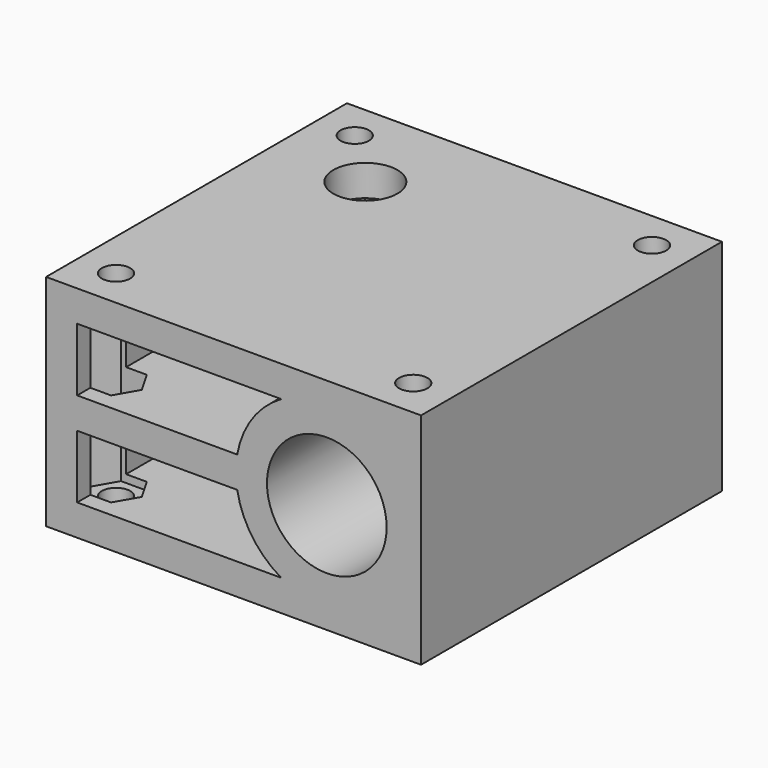
from build123d import *

# Parameters (mm, degrees)
F3_W          = 48.25
F3_H          = 28.25
F3_R          = 7.7
F4_DEPTH      = 24.2
F5_R          = 1.825
F6_DEPTH      = 28.25
F5_R_2        = 4.125
F7_DEPTH      = 28.25
F9_DEPTH      = 13.125
F9_DEPTH_BACK = 9.125


# Not quite as in the source:
# - a feature names something its author has since deleted; it is built from what else it names


with BuildPart() as f4:
    # F3 (on Front) → F4 (new body, symmetric)
    with BuildSketch(Plane.XZ):
        Rectangle(F3_W, F3_H)
        with BuildLine():
            ThreePointArc((23.5277925033, 2), (23.6568686252, 1.0037000824), (23.7, 0))
            ThreePointArc((23.7, 0), (23.6568686252, -1.0037000824), (23.5277925033, -2))
            ThreePointArc((23.5277925033, -2), (22.3372126342, -5.4801491728), (20.125, -8.4186920005))
            Line((20.125, -8.4186920005), (20.125, -10.125))
            Line((20.125, -10.125), (17.8629663994, -10.125))
            ThreePointArc((17.8629663994, -10.125), (15.9935594213, -10.9973398215), (14, -11.5277925033))
            ThreePointArc((14, -11.5277925033), (12, -11.7), (10, -11.5277925033))
            ThreePointArc((10, -11.5277925033), (8.0064405787, -10.9973398215), (6.1370336006, -10.125))
            Line((6.1370336006, -10.125), (-20.125, -10.125))
            Line((-20.125, -10.125), (-20.125, -2))
            Line((-20.125, -2), (-20.125, 2))
            Line((-20.125, 2), (-20.125, 10.125))
            Line((-20.125, 10.125), (6.1370336006, 10.125))
            ThreePointArc((6.1370336006, 10.125), (8.0064405787, 10.9973398215), (10, 11.5277925033))
            ThreePointArc((10, 11.5277925033), (12, 11.7), (14, 11.5277925033))
            ThreePointArc((14, 11.5277925033), (15.9935594213, 10.9973398215), (17.8629663994, 10.125))
            Line((17.8629663994, 10.125), (20.125, 10.125))
            Line((20.125, 10.125), (20.125, 8.4186920005))
            ThreePointArc((20.125, 8.4186920005), (22.3372126342, 5.4801491728), (23.5277925033, 2))
        make_face(mode=Mode.SUBTRACT)
        with BuildLine():
            Line((14, 10.125), (14, 11.5277925033))
            ThreePointArc((14, 11.5277925033), (12, 11.7), (10, 11.5277925033))
            Line((10, 11.5277925033), (10, 10.125))
            Line((10, 10.125), (14, 10.125))
        make_face()
        with BuildLine():
            Line((20.125, 2), (20.125, 8.4186920005))
            ThreePointArc((20.125, 8.4186920005), (19.045826619, 9.3405742466), (17.8629663994, 10.125))
            Line((17.8629663994, 10.125), (14, 10.125))
            Line((14, 10.125), (10, 10.125))
            Line((10, 10.125), (6.1370336006, 10.125))
            ThreePointArc((6.1370336006, 10.125), (2.4024206149, 6.6915222444), (0.4722074967, 2))
            ThreePointArc((0.4722074967, 2), (0.3, 0), (0.4722074967, -2))
            ThreePointArc((0.4722074967, -2), (2.4024206149, -6.6915222444), (6.1370336006, -10.125))
            Line((6.1370336006, -10.125), (10, -10.125))
            Line((10, -10.125), (14, -10.125))
            Line((14, -10.125), (17.8629663994, -10.125))
            ThreePointArc((17.8629663994, -10.125), (19.045826619, -9.3405742466), (20.125, -8.4186920005))
            Line((20.125, -8.4186920005), (20.125, -2))
            Line((20.125, -2), (20.125, 2))
        make_face()
        with Locations((12, 0)):
            Circle(F3_R, mode=Mode.SUBTRACT)
        with BuildLine():
            ThreePointArc((10, -11.5277925033), (12, -11.7), (14, -11.5277925033))
            Line((14, -11.5277925033), (14, -10.125))
            Line((14, -10.125), (10, -10.125))
            Line((10, -10.125), (10, -11.5277925033))
        make_face()
        with BuildLine():
            ThreePointArc((0.4722074967, -2), (0.3, 0), (0.4722074967, 2))
            Line((0.4722074967, 2), (-20.125, 2))
            Line((-20.125, 2), (-20.125, -2))
            Line((-20.125, -2), (0.4722074967, -2))
        make_face()
        with BuildLine():
            ThreePointArc((23.5277925033, -2), (23.6568686252, -1.0037000824), (23.7, 0))
            ThreePointArc((23.7, 0), (23.6568686252, 1.0037000824), (23.5277925033, 2))
            Line((23.5277925033, 2), (20.125, 2))
            Line((20.125, 2), (20.125, -2))
            Line((20.125, -2), (23.5277925033, -2))
        make_face()
        with BuildLine():
            Line((20.125, 2), (23.5277925033, 2))
            ThreePointArc((23.5277925033, 2), (22.3372126342, 5.4801491728), (20.125, 8.4186920005))
            Line((20.125, 8.4186920005), (20.125, 2))
        make_face()
        with BuildLine():
            ThreePointArc((20.125, -8.4186920005), (22.3372126342, -5.4801491728), (23.5277925033, -2))
            Line((23.5277925033, -2), (20.125, -2))
            Line((20.125, -2), (20.125, -8.4186920005))
        make_face()
        with BuildLine():
            Line((14, 10.125), (17.8629663994, 10.125))
            ThreePointArc((17.8629663994, 10.125), (15.9935594213, 10.9973398215), (14, 11.5277925033))
            Line((14, 11.5277925033), (14, 10.125))
        make_face()
        with BuildLine():
            Line((10, 10.125), (10, 11.5277925033))
            ThreePointArc((10, 11.5277925033), (8.0064405787, 10.9973398215), (6.1370336006, 10.125))
            Line((6.1370336006, 10.125), (10, 10.125))
        make_face()
        with BuildLine():
            ThreePointArc((17.8629663994, 10.125), (19.045826619, 9.3405742466), (20.125, 8.4186920005))
            Line((20.125, 8.4186920005), (20.125, 10.125))
            Line((20.125, 10.125), (17.8629663994, 10.125))
        make_face()
        with BuildLine():
            Line((20.125, -10.125), (20.125, -8.4186920005))
            ThreePointArc((20.125, -8.4186920005), (19.045826619, -9.3405742466), (17.8629663994, -10.125))
            Line((17.8629663994, -10.125), (20.125, -10.125))
        make_face()
        with BuildLine():
            ThreePointArc((14, -11.5277925033), (15.9935594213, -10.9973398215), (17.8629663994, -10.125))
            Line((17.8629663994, -10.125), (14, -10.125))
            Line((14, -10.125), (14, -11.5277925033))
        make_face()
        with BuildLine():
            ThreePointArc((6.1370336006, -10.125), (8.0064405787, -10.9973398215), (10, -11.5277925033))
            Line((10, -11.5277925033), (10, -10.125))
            Line((10, -10.125), (6.1370336006, -10.125))
        make_face()
    extrude(amount=F4_DEPTH, both=True)

    # F5 (on face) → F6 (cut)
    with BuildSketch(Plane(origin=(0, 0, -14.125), x_dir=(1, 0, 0), z_dir=(0, 0, -1))):
        with Locations((-19.125, 19.2)):
            Circle(F5_R)
        with Locations((19.125, 19.2)):
            Circle(F5_R)
        with Locations((19.125, -19.2)):
            Circle(F5_R)
        with Locations((-19.125, -19.2)):
            Circle(F5_R)
    extrude(amount=-F6_DEPTH, mode=Mode.SUBTRACT)

    # F5 (on face) → F7 (cut)
    with BuildSketch(Plane(origin=(0, 0, -14.125), x_dir=(1, 0, 0), z_dir=(0, 0, -1))):
        with Locations((-12, -12)):
            Circle(F5_R_2)
    extrude(amount=-F7_DEPTH, mode=Mode.SUBTRACT)

    # F8 (on face) → F9 (cut, two sides)
    with BuildSketch(Plane.XY.offset(2)) as f9_sk:
        Polygon((20.7848820239, -16.325), (17.4651179761, -16.325), (15.8052359522, -19.2), (17.4651179761, -22.075), (20.7848820239, -22.075), (22.4447640478, -19.2), align=None)
        Polygon((17.4651179761, 16.325), (20.7848820239, 16.325), (22.4447640478, 19.2), (20.7848820239, 22.075), (17.4651179761, 22.075), (15.8052359522, 19.2), align=None)
        Polygon((-20.7848820239, 16.325), (-17.4651179761, 16.325), (-15.8052359522, 19.2), (-17.4651179761, 22.075), (-20.7848820239, 22.075), (-22.4447640478, 19.2), align=None)
        Polygon((-17.4651179761, -16.325), (-20.7848820239, -16.325), (-22.4447640478, -19.2), (-20.7848820239, -22.075), (-17.4651179761, -22.075), (-15.8052359522, -19.2), align=None)
    extrude(amount=-F9_DEPTH, mode=Mode.SUBTRACT)
    extrude(f9_sk.sketch, amount=F9_DEPTH_BACK, mode=Mode.SUBTRACT)


solid = f4.part
